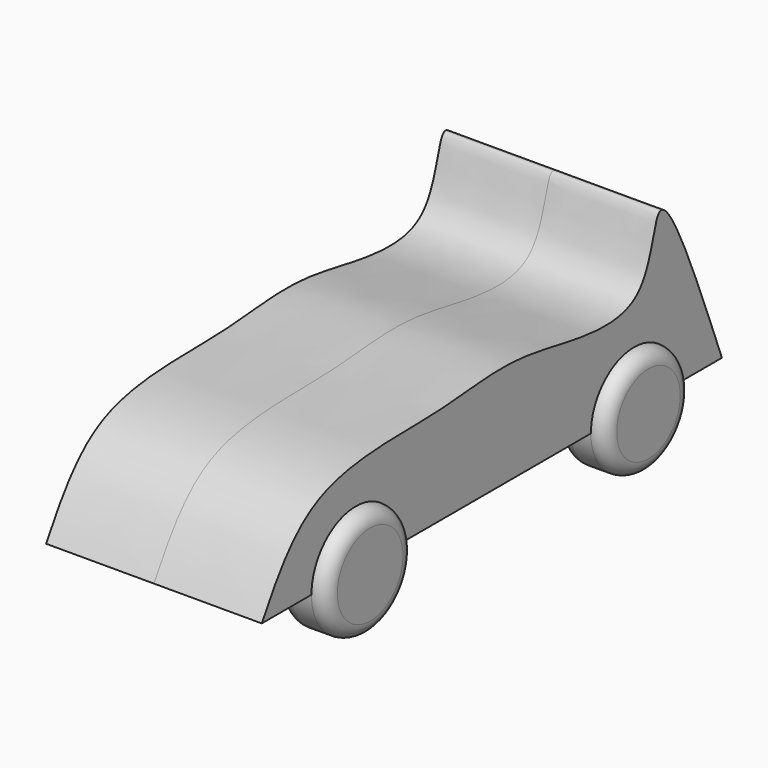
from build123d import *

# Parameters (mm, degrees)
F2_DEPTH    = 19.05
F1_R        = 9.7846675991
F1_R_2      = 9.5471660414
F3_DEPTH    = 21.59
F4_R        = 2.53999
F5_R        = 12.2880612675
F5_R_2      = 12.9742372855
F6_DEPTH    = 12.7
F7_T1_DEPTH = 25.4
F8_R        = 2.54


# Not quite as in the source:
# - a fillet or chamfer that OpenCascade refuses, or shapes differently, is made with other operations: its cross-section is extruded or revolved along the edge and cut away or added
# - a fillet or chamfer is up to 0.001 mm smaller than in the source, because OpenCascade refuses the exact size


with BuildPart() as f2:
    # F0 (on Right) → F2 (new body, symmetric)
    with BuildSketch(Plane.YZ):
        with BuildLine():
            add(Edge.make_bspline(
                [(-39.1218404372, 0), (-35.7499481543, 5.7494593291), (-28.4241148656, 18.2408313222), (1.1758009443, 16.1926491207), (17.7675274811, 20.0311651733), (46.8705269237, 10.6509447037), (47.6094306141, 38.7801853041), (56.7914214175, 14.8319607892), (62.4781595628, 0)],
                knots=[0, 0, 0, 0, 0.1569899924, 0.3410791415, 0.4994622113, 0.67571239, 0.7991566251, 1, 1, 1, 1], degree=3))
            Line((-39.1218404372, 0), (62.4781595628, 0))
        make_face()
    extrude(amount=F2_DEPTH, both=True)

    # F1 (on Right) → F3 (join, symmetric)
    with BuildSketch(Plane.YZ):
        with Locations((-18.3688756078, 0)):
            Circle(F1_R)
        with Locations((43.0892892182, 0)):
            Circle(F1_R_2)
    extrude(amount=F3_DEPTH, both=True)

    # F4 (radius 2.54 in the source; OpenCascade refuses exactly that, so slightly less here)
    f4_edges = [f2.edges().sort_by_distance(p)[0] for p in [
        (21.59, -28.153543, 0),
        (21.59, 33.542123, 0),
        (-21.59, -28.153543, 0),
        (-21.59, 33.542123, 0),
    ]]
    fillet(f4_edges, radius=F4_R)

    # F5 (on Right) → F6 (cut, symmetric)
    with BuildSketch(Plane.YZ):
        with Locations((43.9235679805, 0)):
            Circle(F5_R)
        with Locations((-18.2880014181, 0)):
            Circle(F5_R_2)
    extrude(amount=F6_DEPTH, both=True, mode=Mode.SUBTRACT)

    # F7: chamfer of 25.4 on 2 edges, made by hand

    # F7_s2 → F7_t1 (cut)
    with BuildSketch(Plane.YZ.offset(-12.7)):
        with BuildLine():
            Line((16.0806162314, 0), (34.8454704224, 8.2815816388))
            ThreePointArc((34.8454704224, 8.2815816388), (32.6157253693, 4.8092769929), (31.635506713, 0))
            Line((31.635506713, 0), (16.0806162314, 0))
        make_face()
        with BuildLine():
            Line((10.4769440406, 0), (-8.5626425762, 8.5876788794))
            ThreePointArc((-8.5626425762, 8.5876788794), (-6.2987535844, 4.9587064362), (-5.3137641326, 0))
            Line((-5.3137641326, 0), (10.4769440406, 0))
        make_face()
    extrude(amount=F7_T1_DEPTH, mode=Mode.SUBTRACT)

    # F8
    f8_edges = [f2.edges().sort_by_distance(p)[0] for p in [
        (-12.7, 43.089289, -9.547166),
        (-12.7, -18.368876, -9.784668),
        (12.7, 43.089289, -9.547166),
        (12.7, -18.368876, -9.784668),
    ]]
    fillet(f8_edges, radius=F8_R)


solid = f2.part
